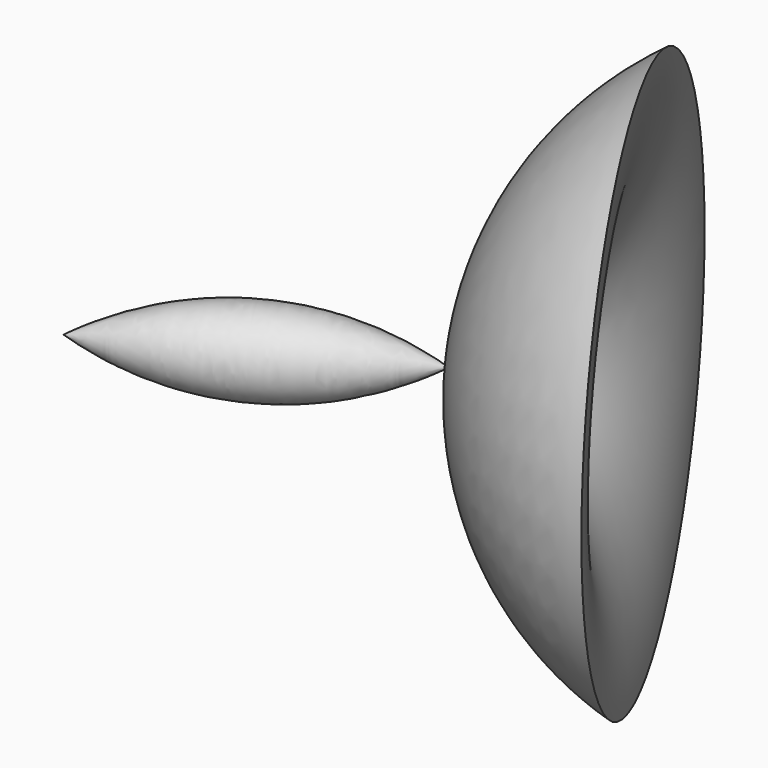
from build123d import *


with BuildPart() as f1:
    # F0 (on Top) → F1 (revolve)
    with BuildSketch(Plane.XY):
        with BuildLine():
            Line((-11.398819356, -6.1144656965), (-0.2266151606, -0.1215591354))
            ThreePointArc((-0.2266151606, -0.1215591354), (-6.614013166, -1.6242061283), (-11.398819356, -6.1144656965))
        make_face()
    revolve(axis=Axis((-5.699409678, -3.0572328482, 0), (0.881223839, 0.4726992126, 0)))


with BuildPart() as f1b:
    # F0 (on Top) → F1, piece 2 (revolve)
    with BuildSketch(Plane.XY):
        with BuildLine():
            ThreePointArc((0.2081435996, 12.5710477015), (-1.6969627469, 6.2855327473), (-0.2072654686, -0.1111797247))
            Line((-0.2072654686, -0.1111797247), (-0.1879491737, -0.1008182286))
            ThreePointArc((-0.1879491737, -0.1008182286), (1.7044193602, 6.1821542047), (0.2081435996, 12.5710477015))
        make_face()
    revolve(axis=Axis((-5.699409678, -3.0572328482, 0), (0.881223839, 0.4726992126, 0)))


solid = Compound([f1.part, f1b.part])
